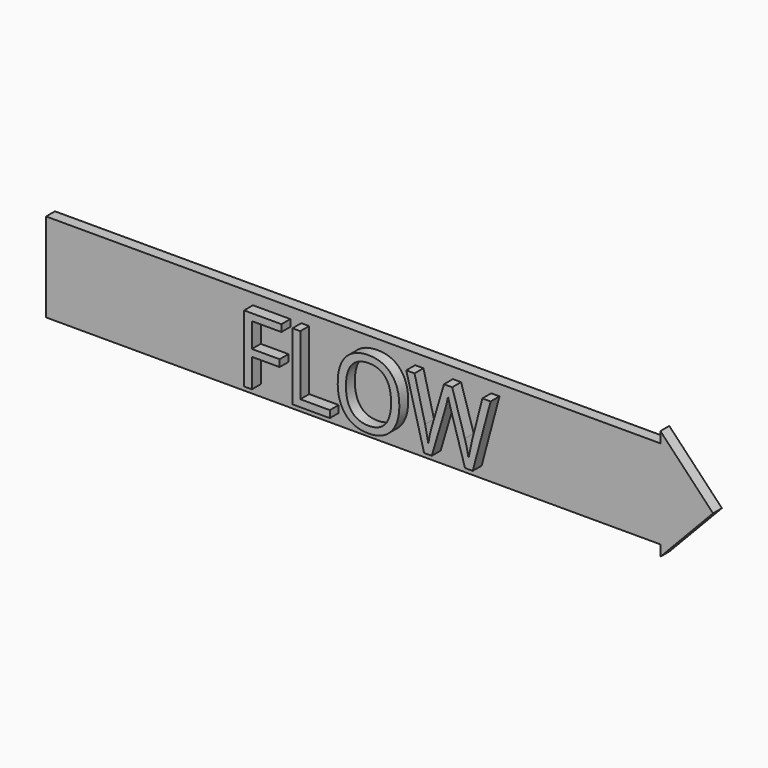
from build123d import *

# Parameters (mm, degrees)
F1_DEPTH     = 25
F2_TEXT_SIZE = 210.9920088616
F3_DEPTH     = 25


# Not quite as in the source:
# - Text() gives the source's letters only with a copy of the font that has no kerning and outlines rounded to 1/6400 em; it was checked with that copy


with BuildPart() as f1:
    # F0 (on Front) → F1 (new body)
    with BuildSketch(Plane.XZ):
        Polygon((0, 100), (0, 0), (1500, 0), (1381.6199234133, 124.3958962734), (1381.6199234133, 100), align=None)
        Polygon((1500, 0), (0, 0), (0, -100), (1381.6199234133, -100), (1381.6199234133, -124.3958962734), align=None)
    extrude(amount=-F1_DEPTH)

    # F2 (on Front) → F3 (join)
    with BuildSketch(Plane.XZ):
        with Locations((444.6024596691, -75.1736909151)):
            Text('FLOW', F2_TEXT_SIZE, font='Open Sans', text_align=(TextAlign.LEFT, TextAlign.BOTTOM))
    extrude(amount=F3_DEPTH)


solid = f1.part
